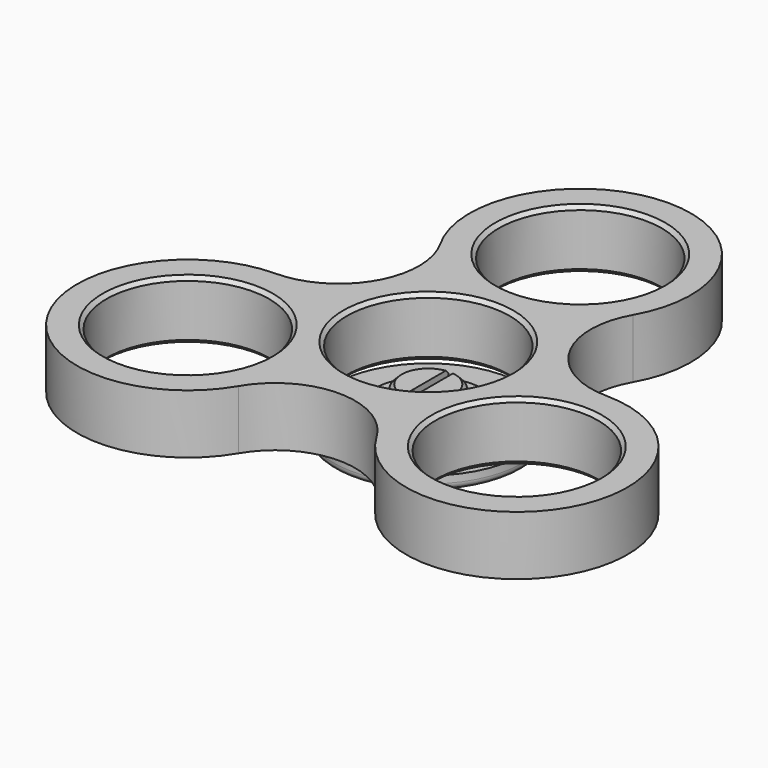
from build123d import *

# Parameters (mm, degrees)
F0_R      = 11.15
F1_DEPTH  = 8.1
F2_SIZE   = 0.5
F3_R      = 4.14
F4_DEPTH  = 3
F5_R      = 7.5
F6_DEPTH  = 1.25
F7_R      = 13
F8_DEPTH  = 2
F9_R      = 1
F10_SIZE  = 0.5
F11_W     = 1
F11_H     = 10.2475439198
F12_DEPTH = 2


# Not quite as in the source:
# - a feature names something its author has since deleted; it is built from what else it names


with BuildPart() as f1:
    # F0 (on Top) → F1 (new body)
    with BuildSketch(Plane.XY):
        with BuildLine():
            ThreePointArc((22.6266893771, 2.1495550685), (13.2144351026, 7.6293576707), (13.1749139786, 18.5205102804))
            ThreePointArc((13.1749139786, 18.5205102804), (0, 41.1500919302), (-13.1749139786, 18.5205102804))
            ThreePointArc((-13.1749139786, 18.5205102804), (-13.2144351026, 7.6293576707), (-22.6266893771, 2.1495550685))
            ThreePointArc((-22.6266893771, 2.1495550685), (-35.6370249735, -20.5750459546), (-9.4517753985, -20.6700653278))
            ThreePointArc((-9.4517753985, -20.6700653278), (0, -15.2587153203), (9.4517753985, -20.6700653278))
            ThreePointArc((9.4517753985, -20.6700653278), (35.6370249736, -20.5750459545), (22.6266893771, 2.1495550685))
        make_face()
        with Locations((-22.5167401062, -13.0000459546)):
            Circle(F0_R, mode=Mode.SUBTRACT)
        Circle(F0_R, mode=Mode.SUBTRACT)
        with Locations((22.5167401062, -13.0000459546)):
            Circle(F0_R, mode=Mode.SUBTRACT)
        with Locations((0, 26.0000919302)):
            Circle(F0_R, mode=Mode.SUBTRACT)
    extrude(amount=F1_DEPTH)

    # F2
    f2_edges = [f1.edges().sort_by_distance(p)[0] for p in [
        (-11.15, 0, 8.1),
        (-11.15, 26.000092, 8.1),
        (-11.15, 26.000092, 0),
        (-11.15, 0, 0),
        (11.36674, -13.000046, 8.1),
        (-33.66674, -13.000046, 8.1),
        (-33.66674, -13.000046, 0),
        (11.36674, -13.000046, 0),
    ]]
    chamfer(f2_edges, length=F2_SIZE)


with BuildPart() as f4:
    # F3 (on Top) → F4 (new body)
    with BuildSketch(Plane.XY):
        Circle(F3_R)
    extrude(amount=F4_DEPTH)

    # F5 (on face) → F6 (join)
    with BuildSketch(Plane(origin=(0, 0, 0), x_dir=(1, 0, 0), z_dir=(0, 0, -1))):
        Circle(F5_R)
    extrude(amount=F6_DEPTH)

    # F7 (on face) → F8 (join)
    with BuildSketch(Plane(origin=(0, 0, -1.25), x_dir=(1, 0, 0), z_dir=(0, 0, -1))):
        Circle(F7_R)
    extrude(amount=F8_DEPTH)

    # F9
    f9_edges = [f4.edges().sort_by_distance(p)[0] for p in [
        (-13, 0, -3.25),
    ]]
    fillet(f9_edges, radius=F9_R)

    # F10
    f10_edges = [f4.edges().sort_by_distance(p)[0] for p in [
        (-4.14, 0, 3),
    ]]
    chamfer(f10_edges, length=F10_SIZE)

    # F11 (on face) → F12 (cut)
    with BuildSketch(Plane.XY.offset(3)):
        with Locations((0, 0.1778125297)):
            Rectangle(F11_W, F11_H)
    extrude(amount=-F12_DEPTH, mode=Mode.SUBTRACT)


solid = Compound([f1.part, f4.part])
